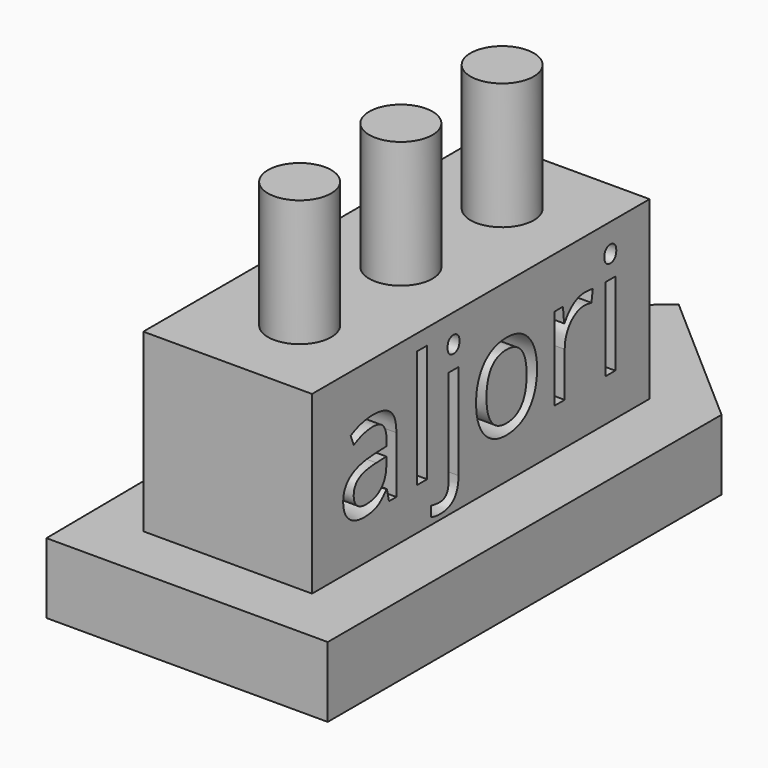
from build123d import *

# Parameters (mm, degrees)
F1_DEPTH     = 10
F2_W         = 24
F2_H         = 60
F3_DEPTH     = 25
F4_R         = 4.5
F5_DEPTH     = 18
F6_TEXT_SIZE = 22.0323731709
F7_DEPTH     = 5
F8_TEXT_SIZE = 15.343974034
F9_DEPTH     = 5


# Not quite as in the source:
# - Text() gives the source's letters only with a copy of the font that has no kerning and outlines rounded to 1/6400 em; it was checked with that copy


with BuildPart() as f1:
    # F0 (on Top) → F1 (new body)
    with BuildSketch(Plane.XY):
        Polygon((20, -28.5289473832), (20, 41.4710526168), (-0.3258111726, 59.2435425992), (-20.6516223452, 41.4710526168), (-20, -28.5289473832), align=None)
    extrude(amount=F1_DEPTH)

    # F2 (on face) → F3 (join)
    with BuildSketch(Plane.XY.offset(10)):
        with Locations((-0.6326579497, 9.4710526168)):
            Rectangle(F2_W, F2_H)
    extrude(amount=F3_DEPTH)

    # F4 (on face) → F5 (join)
    with BuildSketch(Plane.XY.offset(35)):
        with Locations((0, 27.4710526168)):
            Circle(F4_R)
        with Locations((0, 9.4710526168)):
            Circle(F4_R)
        with Locations((0, -8.5289473832)):
            Circle(F4_R)
    extrude(amount=F5_DEPTH)

    # F6 (on face) → F7 (cut)
    with BuildSketch(Plane.YZ.offset(11.3673420503)):
        with Locations((-16.0049460828, 16.0049479455)):
            Text('aljori', F6_TEXT_SIZE, font='Open Sans', text_align=(TextAlign.LEFT, TextAlign.BOTTOM))
    extrude(amount=-F7_DEPTH, mode=Mode.SUBTRACT)

    # F8 (on face) → F9 (cut)
    with BuildSketch(Plane(origin=(-12.6326579497, 0, 0), x_dir=(0, -1, 0), z_dir=(-1, 0, 0))):
        with Locations((-35.2675393224, 16.8547648937)):
            Text('shaden', F8_TEXT_SIZE, font='Open Sans', text_align=(TextAlign.LEFT, TextAlign.BOTTOM))
    extrude(amount=-F9_DEPTH, mode=Mode.SUBTRACT)


solid = f1.part
